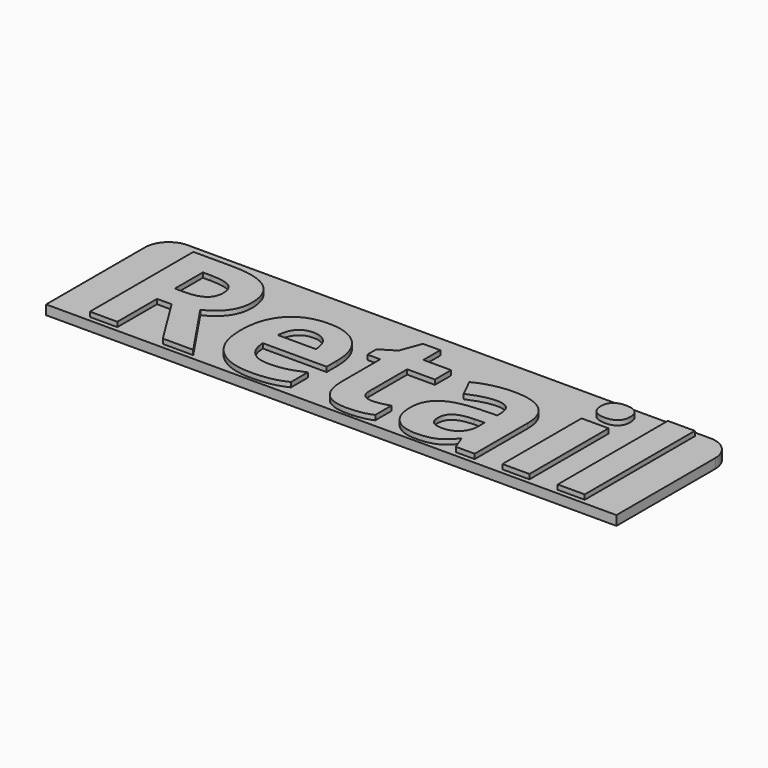
from build123d import *

# Parameters (mm, degrees)
F0_W         = 120
F0_H         = 31
F1_DEPTH     = 2
F2_TEXT_SIZE = 38.1138000108
F3_DEPTH     = 1
F4_R         = 5


# Not quite as in the source:
# - Text() gives the source's letters only with a copy of the font that has no kerning and outlines rounded to 1/6400 em; it was checked with that copy


with BuildPart() as f1:
    # F0 (on Top) → F1 (new body)
    with BuildSketch(Plane.XY):
        Rectangle(F0_W, F0_H)
    extrude(amount=F1_DEPTH)

    # F2 (on face) → F3 (join)
    with BuildSketch(Plane.XY.offset(2)):
        with Locations((-55, -14.5)):
            Text('Retail', F2_TEXT_SIZE, font='Open Sans', font_style=FontStyle.BOLD, text_align=(TextAlign.LEFT, TextAlign.BOTTOM))
    extrude(amount=F3_DEPTH)

    # F4
    f4_edges = [f1.edges().sort_by_distance(p)[0] for p in [
        (-60, 15.5, 1),
        (60, 15.5, 1),
    ]]
    fillet(f4_edges, radius=F4_R)


solid = f1.part
